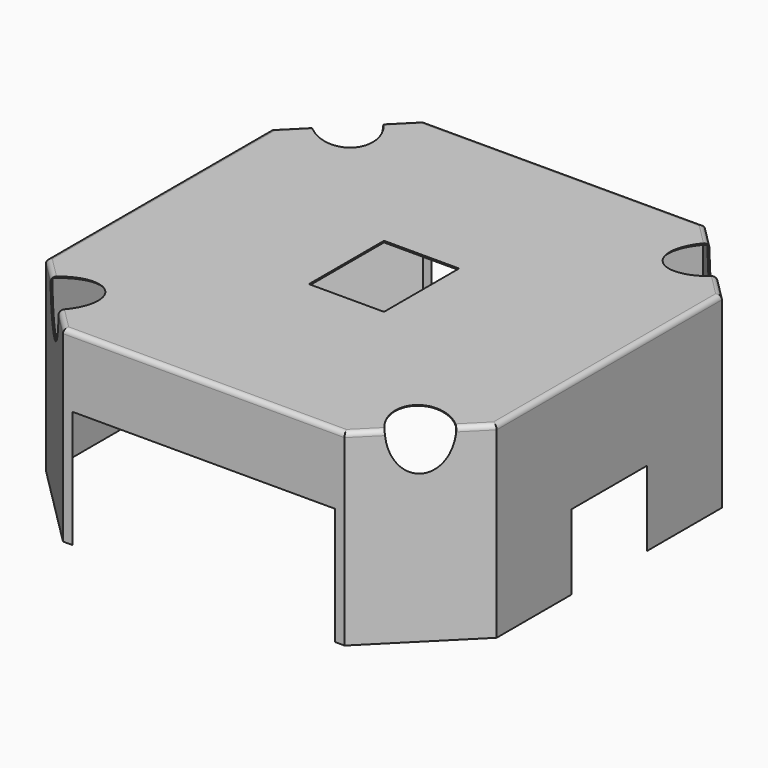
from build123d import *

# Parameters (mm, degrees)
F1_DEPTH       = 240
F2_SIZE        = 90
F3_T           = -1.6
F10_R          = 30
F12_DEPTH      = 78
F11_R          = 30
F13_DEPTH      = 82
F8_R           = 30
F14_DEPTH      = 153
F9_R           = 30
F15_DEPTH      = 141
F17_DEPTH      = 688
F18_W          = 80
F18_H          = 100
F19_DEPTH      = 25
F20_T1_DEPTH   = 325
F20_T3_DEPTH   = 58.6396103068
F20_T5_DEPTH   = 58.6396103068
F20_T7_DEPTH   = 58.6396103068
F20_T9_DEPTH   = 58.6396103068
F20_T11_DEPTH  = 325
F20_T13_DEPTH  = 58.6396103068
F20_T15_DEPTH  = 58.6396103068
F20_T17_DEPTH  = 134.1651513899
F20_T19_DEPTH  = 280
F20_T21_DEPTH  = 89.1651513899
F20_T23_DEPTH  = 100
F20_T29_DEPTH  = 134.1651513899
F20_T33_DEPTH  = 289.1651513899
F20_T40_DEPTH  = 289.1651513899
F20_T44_DEPTH  = 134.1651513899
F20_T51_DEPTH  = 89.1651513899
F20_T55_DEPTH  = 109.1651513899
F20_T62_DEPTH  = 109.1651513899
F20_T66_DEPTH  = 89.1651513899
F20_T73_DEPTH  = 89.1651513899
F20_T77_DEPTH  = 109.1651513899
F20_T84_DEPTH  = 89.1651513899
F20_T88_DEPTH  = 109.1651513899
F20_T95_DEPTH  = 289.1651513899
F20_T99_DEPTH  = 134.1651513899
F20_T106_DEPTH = 134.1651513899
F20_T110_DEPTH = 289.1651513899


# Not quite as in the source:
# - a fillet or chamfer that OpenCascade refuses, or shapes differently, is made with other operations: its cross-section is extruded or revolved along the edge and cut away or added


with BuildPart() as f1:
    # F0 (on Front) → F1 (new body, symmetric)
    with BuildSketch(Plane.XZ):
        Polygon((140, -100), (240, -100), (240, 100), (-240, 100), (-240, -100), (-140, -100), (-140, 25), (140, 25), align=None)
    extrude(amount=F1_DEPTH, both=True)

    # F2
    f2_edges = [f1.edges().sort_by_distance(p)[0] for p in [
        (240, -240, 0),
        (240, 240, 0),
        (-240, 240, 0),
        (-240, -240, 0),
    ]]
    chamfer(f2_edges, length=F2_SIZE)

    # F3
    f3_openings = [f1.faces().sort_by_distance(p)[0] for p in [
        (185.93985, 0, -100),
        (-185.93985, 0, -100),
        (0, 0, 25),
        (140, 0, -37.5),
        (-140, 0, -37.5),
    ]]
    offset(amount=F3_T, openings=f3_openings)

    # F10 (on face) → F12 (cut)
    with BuildSketch(Plane(origin=(-132.8553390593, 132.8553390593, 187.8858223314), x_dir=(0.8660254038, 0.2886751346, 0.4082482905), z_dir=(0.5, -0.5, -0.7071067812))):
        with Locations((-71.7584734456, -101.4818063619)):
            Circle(F10_R)
    extrude(amount=F12_DEPTH, mode=Mode.SUBTRACT)

    # F11 (on face) → F13 (cut)
    with BuildSketch(Plane(origin=(-132.8553390593, -132.8553390593, 187.8858223314), x_dir=(0.8660254038, -0.2886751346, 0.4082482905), z_dir=(-0.5, -0.5, 0.7071067812))):
        with Locations((-71.7584734456, -101.4818063619)):
            Circle(F11_R)
    extrude(amount=-F13_DEPTH, mode=Mode.SUBTRACT)

    # F8 (on face) → F14 (cut)
    with BuildSketch(Plane(origin=(132.8553390593, -132.8553390593, 187.8858223314), x_dir=(0.8660254038, 0.2886751346, -0.4082482905), z_dir=(0.5, -0.5, 0.7071067812))):
        with Locations((71.7584734456, -101.4818063619)):
            Circle(F8_R)
    extrude(amount=-F14_DEPTH, mode=Mode.SUBTRACT)

    # F9 (on face) → F15 (cut)
    with BuildSketch(Plane(origin=(132.8553390593, 132.8553390593, 187.8858223314), x_dir=(0.8660254038, -0.2886751346, -0.4082482905), z_dir=(-0.5, -0.5, -0.7071067812))):
        with Locations((71.7584734456, -101.4818063619)):
            Circle(F9_R)
    extrude(amount=F15_DEPTH, mode=Mode.SUBTRACT)

    # F16 (on face) → F17 (cut)
    with BuildSketch(Plane(origin=(-240, 0, 0), x_dir=(0, -1, 0), z_dir=(-1, 0, 0))):
        Polygon((-50, -20), (-50, -100), (0, -100), (50, -100), (50, -20), align=None)
    extrude(amount=-F17_DEPTH, mode=Mode.SUBTRACT)

    # F18 (on face) → F19 (cut)
    with BuildSketch(Plane.XY.offset(100)):
        Rectangle(F18_W, F18_H)
    extrude(amount=-F19_DEPTH, mode=Mode.SUBTRACT)

    # F20: fillet of radius 5 on 24 edges, made by hand

    # F20_s2 → F20_t1 (cut)
    with BuildSketch(Plane.YZ.offset(-162.5)):
        with BuildLine():
            ThreePointArc((235, 100), (238.5355339059, 98.5355339059), (240, 95))
            Line((240, 95), (240, 100))
            Line((240, 100), (235, 100))
        make_face()
        with BuildLine():
            ThreePointArc((-240, 95), (-238.5355339059, 98.5355339059), (-235, 100))
            Line((-235, 100), (-240, 100))
            Line((-240, 100), (-240, 95))
        make_face()
    extrude(amount=F20_T1_DEPTH, mode=Mode.SUBTRACT)

    # F20_s4 → F20_t3 (cut)
    with BuildSketch(Plane(origin=(12.3743686708, 12.3743686708, 0), x_dir=(0, 0, 1), z_dir=(0.7071067812, 0.7071067812, 0))):
        with BuildLine():
            ThreePointArc((100, -270.7716446628), (98.5355339059, -274.3071785687), (95, -275.7716446628))
            Line((95, -275.7716446628), (100, -275.7716446628))
            Line((100, -275.7716446628), (100, -270.7716446628))
        make_face()
        with BuildLine():
            ThreePointArc((95, 275.7716446628), (98.5355339059, 274.3071785687), (100, 270.7716446628))
            Line((100, 270.7716446628), (100, 275.7716446628))
            Line((100, 275.7716446628), (95, 275.7716446628))
        make_face()
    extrude(amount=F20_T3_DEPTH, mode=Mode.SUBTRACT)

    # F20_s6 → F20_t5 (cut)
    with BuildSketch(Plane(origin=(-12.3743686708, 12.3743686708, 0), x_dir=(0, 0, 1), z_dir=(-0.7071067812, 0.7071067812, 0))):
        with BuildLine():
            ThreePointArc((100, 270.7716446628), (98.5355339059, 274.3071785687), (95, 275.7716446628))
            Line((95, 275.7716446628), (100, 275.7716446628))
            Line((100, 275.7716446628), (100, 270.7716446628))
        make_face()
    extrude(amount=F20_T5_DEPTH, mode=Mode.SUBTRACT)

    # F20_s8 → F20_t7 (cut)
    with BuildSketch(Plane(origin=(53.8388347648, -53.8388347648, 0), x_dir=(0, 0, 1), z_dir=(-0.7071067812, 0.7071067812, 0))):
        with BuildLine():
            ThreePointArc((100, 270.7716446628), (98.5355339059, 274.3071785687), (95, 275.7716446628))
            Line((95, 275.7716446628), (100, 275.7716446628))
            Line((100, 275.7716446628), (100, 270.7716446628))
        make_face()
    extrude(amount=F20_T7_DEPTH, mode=Mode.SUBTRACT)

    # F20_s10 → F20_t9 (cut)
    with BuildSketch(Plane(origin=(-53.8388347648, -53.8388347648, 0), x_dir=(0, 0, 1), z_dir=(0.7071067812, 0.7071067812, 0))):
        with BuildLine():
            ThreePointArc((100, -270.7716446628), (98.5355339059, -274.3071785687), (95, -275.7716446628))
            Line((95, -275.7716446628), (100, -275.7716446628))
            Line((100, -275.7716446628), (100, -270.7716446628))
        make_face()
        with BuildLine():
            ThreePointArc((95, 275.7716446628), (98.5355339059, 274.3071785687), (100, 270.7716446628))
            Line((100, 270.7716446628), (100, 275.7716446628))
            Line((100, 275.7716446628), (95, 275.7716446628))
        make_face()
    extrude(amount=F20_T9_DEPTH, mode=Mode.SUBTRACT)

    # F20_s12 → F20_t11 (cut)
    with BuildSketch(Plane.XZ.offset(-162.5)):
        with BuildLine():
            ThreePointArc((-235, 100), (-238.5355339059, 98.5355339059), (-240, 95))
            Line((-240, 95), (-240, 100))
            Line((-240, 100), (-235, 100))
        make_face()
        with BuildLine():
            ThreePointArc((235, 100), (238.5355339059, 98.5355339059), (240, 95))
            Line((240, 95), (240, 100))
            Line((240, 100), (235, 100))
        make_face()
    extrude(amount=F20_T11_DEPTH, mode=Mode.SUBTRACT)

    # F20_s14 → F20_t13 (cut)
    with BuildSketch(Plane(origin=(-53.8388347648, 53.8388347648, 0), x_dir=(0, 0, 1), z_dir=(0.7071067812, -0.7071067812, 0))):
        with BuildLine():
            ThreePointArc((100, 270.7716446628), (98.5355339059, 274.3071785687), (95, 275.7716446628))
            Line((95, 275.7716446628), (100, 275.7716446628))
            Line((100, 275.7716446628), (100, 270.7716446628))
        make_face()
    extrude(amount=F20_T13_DEPTH, mode=Mode.SUBTRACT)

    # F20_s16 → F20_t15 (cut)
    with BuildSketch(Plane(origin=(12.3743686708, -12.3743686708, 0), x_dir=(0, 0, 1), z_dir=(0.7071067812, -0.7071067812, 0))):
        with BuildLine():
            ThreePointArc((100, 270.7716446628), (98.5355339059, 274.3071785687), (95, 275.7716446628))
            Line((95, 275.7716446628), (100, 275.7716446628))
            Line((100, 275.7716446628), (100, 270.7716446628))
        make_face()
    extrude(amount=F20_T15_DEPTH, mode=Mode.SUBTRACT)

    # F20_s18 → F20_t17 (cut)
    with BuildSketch(Plane.XY.offset(-109.1651513899)):
        with BuildLine():
            ThreePointArc((140, -240), (141.666060556, -238.817424305), (143.666060556, -238.4))
            Line((143.666060556, -238.4), (140, -238.4))
            Line((140, -238.4), (140, -240))
        make_face()
        with BuildLine():
            ThreePointArc((-140, -240), (-141.666060556, -238.817424305), (-143.666060556, -238.4))
            Line((-143.666060556, -238.4), (-140, -238.4))
            Line((-140, -238.4), (-140, -240))
        make_face()
        with BuildLine():
            ThreePointArc((143.666060556, 240), (141.666060556, 239.582575695), (140, 238.4))
            Line((140, 238.4), (140, 240))
            Line((140, 240), (143.666060556, 240))
        make_face()
        with BuildLine():
            ThreePointArc((-143.666060556, 240), (-141.666060556, 239.582575695), (-140, 238.4))
            Line((-140, 238.4), (-140, 240))
            Line((-140, 240), (-143.666060556, 240))
        make_face()
    extrude(amount=F20_T17_DEPTH, mode=Mode.SUBTRACT)

    # F20_s20 → F20_t19 (cut)
    with BuildSketch(Plane.YZ.offset(-140)):
        with BuildLine():
            ThreePointArc((-240, 25), (-238.817424305, 26.666060556), (-238.4, 28.666060556))
            Line((-238.4, 28.666060556), (-238.4, 25))
            Line((-238.4, 25), (-240, 25))
        make_face()
        with BuildLine():
            ThreePointArc((240, 28.666060556), (239.582575695, 26.666060556), (238.4, 25))
            Line((238.4, 25), (240, 25))
            Line((240, 25), (240, 28.666060556))
        make_face()
    extrude(amount=F20_T19_DEPTH, mode=Mode.SUBTRACT)

    # F20_s22 → F20_t21 (cut)
    with BuildSketch(Plane.XY.offset(-109.1651513899)):
        with BuildLine():
            ThreePointArc((-238.4, -53.666060556), (-238.817424305, -51.666060556), (-240, -50))
            Line((-240, -50), (-238.4, -50))
            Line((-238.4, -50), (-238.4, -53.666060556))
        make_face()
        with BuildLine():
            ThreePointArc((-238.4, 53.666060556), (-238.817424305, 51.666060556), (-240, 50))
            Line((-240, 50), (-238.4, 50))
            Line((-238.4, 50), (-238.4, 53.666060556))
        make_face()
        with BuildLine():
            ThreePointArc((240, -50), (238.817424305, -51.666060556), (238.4, -53.666060556))
            Line((238.4, -53.666060556), (238.4, -50))
            Line((238.4, -50), (240, -50))
        make_face()
        with BuildLine():
            ThreePointArc((238.4, 53.666060556), (238.817424305, 51.666060556), (240, 50))
            Line((240, 50), (238.4, 50))
            Line((238.4, 50), (238.4, 53.666060556))
        make_face()
    extrude(amount=F20_T21_DEPTH, mode=Mode.SUBTRACT)

    # F20_s24 → F20_t23 (cut)
    with BuildSketch(Plane.XZ.offset(-50)):
        with BuildLine():
            ThreePointArc((-238.4, -16.333939444), (-238.817424305, -18.333939444), (-240, -20))
            Line((-240, -20), (-238.4, -20))
            Line((-238.4, -20), (-238.4, -16.333939444))
        make_face()
        with BuildLine():
            ThreePointArc((238.4, -16.333939444), (238.817424305, -18.333939444), (240, -20))
            Line((240, -20), (238.4, -20))
            Line((238.4, -20), (238.4, -16.333939444))
        make_face()
    extrude(amount=F20_T23_DEPTH, mode=Mode.SUBTRACT)


with BuildPart() as f20_tool27:
    # F20_s28 → F20_t29 (new body)
    with BuildSketch(Plane.XY.offset(34.1651513899)):
        with BuildLine():
            ThreePointArc((140, -240), (141.666060556, -238.817424305), (143.666060556, -238.4))
            Line((143.666060556, -238.4), (140, -238.4))
            Line((140, -238.4), (140, -240))
        make_face()
    extrude(amount=-F20_T29_DEPTH)

    split(bisect_by=Plane.XY.offset(25), keep=Keep.TOP)


with BuildPart() as f20_tool31:
    # F20_s32 → F20_t33 (new body)
    with BuildSketch(Plane.YZ.offset(-140)):
        with BuildLine():
            ThreePointArc((-240, 25), (-238.817424305, 26.666060556), (-238.4, 28.666060556))
            Line((-238.4, 28.666060556), (-238.4, 25))
            Line((-238.4, 25), (-240, 25))
        make_face()
    extrude(amount=F20_T33_DEPTH)

    split(bisect_by=Plane.YZ.offset(140), keep=Keep.TOP)


with BuildPart() as f20_tool27_1:
    add(f20_tool27.part)

    # F20_t35: intersect F20_tool31
    add(f20_tool31.part, mode=Mode.INTERSECT)


with BuildPart() as f1_1:
    add(f1.part)

    # F20_t25: cut F20_tool27
    add(f20_tool27_1.part, mode=Mode.SUBTRACT)


with BuildPart() as f20_tool38:
    # F20_s39 → F20_t40 (new body)
    with BuildSketch(Plane.YZ.offset(-149.1651513899)):
        with BuildLine():
            ThreePointArc((-240, 25), (-238.817424305, 26.666060556), (-238.4, 28.666060556))
            Line((-238.4, 28.666060556), (-238.4, 25))
            Line((-238.4, 25), (-240, 25))
        make_face()
    extrude(amount=F20_T40_DEPTH)

    split(bisect_by=Plane.YZ.offset(-140), keep=Keep.BOTTOM)


with BuildPart() as f20_tool42:
    # F20_s43 → F20_t44 (new body)
    with BuildSketch(Plane.XY.offset(-100)):
        with BuildLine():
            ThreePointArc((-140, -240), (-141.666060556, -238.817424305), (-143.666060556, -238.4))
            Line((-143.666060556, -238.4), (-140, -238.4))
            Line((-140, -238.4), (-140, -240))
        make_face()
    extrude(amount=F20_T44_DEPTH)

    split(bisect_by=Plane.XY.offset(25), keep=Keep.TOP)


with BuildPart() as f20_tool38_1:
    add(f20_tool38.part)

    # F20_t46: intersect F20_tool42
    add(f20_tool42.part, mode=Mode.INTERSECT)


with BuildPart() as f1_2:
    add(f1_1.part)

    # F20_t36: cut F20_tool38
    add(f20_tool38_1.part, mode=Mode.SUBTRACT)


with BuildPart() as f20_tool49:
    # F20_s50 → F20_t51 (new body)
    with BuildSketch(Plane.XY.offset(-100)):
        with BuildLine():
            ThreePointArc((-238.4, -53.666060556), (-238.817424305, -51.666060556), (-240, -50))
            Line((-240, -50), (-238.4, -50))
            Line((-238.4, -50), (-238.4, -53.666060556))
        make_face()
    extrude(amount=F20_T51_DEPTH)

    split(bisect_by=Plane.XY.offset(-20), keep=Keep.TOP)


with BuildPart() as f20_tool53:
    # F20_s54 → F20_t55 (new body)
    with BuildSketch(Plane.XZ.offset(59.1651513899)):
        with BuildLine():
            ThreePointArc((-238.4, -16.333939444), (-238.817424305, -18.333939444), (-240, -20))
            Line((-240, -20), (-238.4, -20))
            Line((-238.4, -20), (-238.4, -16.333939444))
        make_face()
    extrude(amount=-F20_T55_DEPTH)

    split(bisect_by=Plane.XZ.offset(50), keep=Keep.TOP)


with BuildPart() as f20_tool49_1:
    add(f20_tool49.part)

    # F20_t57: intersect F20_tool53
    add(f20_tool53.part, mode=Mode.INTERSECT)


with BuildPart() as f1_3:
    add(f1_2.part)

    # F20_t47: cut F20_tool49
    add(f20_tool49_1.part, mode=Mode.SUBTRACT)


with BuildPart() as f20_tool60:
    # F20_s61 → F20_t62 (new body)
    with BuildSketch(Plane.XZ.offset(50)):
        with BuildLine():
            ThreePointArc((-238.4, -16.333939444), (-238.817424305, -18.333939444), (-240, -20))
            Line((-240, -20), (-238.4, -20))
            Line((-238.4, -20), (-238.4, -16.333939444))
        make_face()
    extrude(amount=-F20_T62_DEPTH)

    split(bisect_by=Plane.XZ.offset(-50), keep=Keep.BOTTOM)


with BuildPart() as f20_tool64:
    # F20_s65 → F20_t66 (new body)
    with BuildSketch(Plane.XY.offset(-10.8348486101)):
        with BuildLine():
            ThreePointArc((-238.4, 53.666060556), (-238.817424305, 51.666060556), (-240, 50))
            Line((-240, 50), (-238.4, 50))
            Line((-238.4, 50), (-238.4, 53.666060556))
        make_face()
    extrude(amount=-F20_T66_DEPTH)

    split(bisect_by=Plane.XY.offset(-20), keep=Keep.TOP)


with BuildPart() as f20_tool60_1:
    add(f20_tool60.part)

    # F20_t68: intersect F20_tool64
    add(f20_tool64.part, mode=Mode.INTERSECT)


with BuildPart() as f1_4:
    add(f1_3.part)

    # F20_t58: cut F20_tool60
    add(f20_tool60_1.part, mode=Mode.SUBTRACT)


with BuildPart() as f20_tool71:
    # F20_s72 → F20_t73 (new body)
    with BuildSketch(Plane.XY.offset(-10.8348486101)):
        with BuildLine():
            ThreePointArc((240, -50), (238.817424305, -51.666060556), (238.4, -53.666060556))
            Line((238.4, -53.666060556), (238.4, -50))
            Line((238.4, -50), (240, -50))
        make_face()
    extrude(amount=-F20_T73_DEPTH)

    split(bisect_by=Plane.XY.offset(-20), keep=Keep.TOP)


with BuildPart() as f20_tool75:
    # F20_s76 → F20_t77 (new body)
    with BuildSketch(Plane.XZ.offset(-50)):
        with BuildLine():
            ThreePointArc((238.4, -16.333939444), (238.817424305, -18.333939444), (240, -20))
            Line((240, -20), (238.4, -20))
            Line((238.4, -20), (238.4, -16.333939444))
        make_face()
    extrude(amount=F20_T77_DEPTH)

    split(bisect_by=Plane.XZ.offset(50), keep=Keep.TOP)


with BuildPart() as f20_tool71_1:
    add(f20_tool71.part)

    # F20_t79: intersect F20_tool75
    add(f20_tool75.part, mode=Mode.INTERSECT)


with BuildPart() as f1_5:
    add(f1_4.part)

    # F20_t69: cut F20_tool71
    add(f20_tool71_1.part, mode=Mode.SUBTRACT)


with BuildPart() as f20_tool82:
    # F20_s83 → F20_t84 (new body)
    with BuildSketch(Plane.XY.offset(-100)):
        with BuildLine():
            ThreePointArc((238.4, 53.666060556), (238.817424305, 51.666060556), (240, 50))
            Line((240, 50), (238.4, 50))
            Line((238.4, 50), (238.4, 53.666060556))
        make_face()
    extrude(amount=F20_T84_DEPTH)

    split(bisect_by=Plane.XY.offset(-20), keep=Keep.TOP)


with BuildPart() as f20_tool86:
    # F20_s87 → F20_t88 (new body)
    with BuildSketch(Plane.XZ.offset(-59.1651513899)):
        with BuildLine():
            ThreePointArc((238.4, -16.333939444), (238.817424305, -18.333939444), (240, -20))
            Line((240, -20), (238.4, -20))
            Line((238.4, -20), (238.4, -16.333939444))
        make_face()
    extrude(amount=F20_T88_DEPTH)

    split(bisect_by=Plane.XZ.offset(-50), keep=Keep.BOTTOM)


with BuildPart() as f20_tool82_1:
    add(f20_tool82.part)

    # F20_t90: intersect F20_tool86
    add(f20_tool86.part, mode=Mode.INTERSECT)


with BuildPart() as f1_6:
    add(f1_5.part)

    # F20_t80: cut F20_tool82
    add(f20_tool82_1.part, mode=Mode.SUBTRACT)


with BuildPart() as f20_tool93:
    # F20_s94 → F20_t95 (new body)
    with BuildSketch(Plane.YZ.offset(-149.1651513899)):
        with BuildLine():
            ThreePointArc((240, 28.666060556), (239.582575695, 26.666060556), (238.4, 25))
            Line((238.4, 25), (240, 25))
            Line((240, 25), (240, 28.666060556))
        make_face()
    extrude(amount=F20_T95_DEPTH)

    split(bisect_by=Plane.YZ.offset(-140), keep=Keep.BOTTOM)


with BuildPart() as f20_tool97:
    # F20_s98 → F20_t99 (new body)
    with BuildSketch(Plane.XY.offset(-100)):
        with BuildLine():
            ThreePointArc((-143.666060556, 240), (-141.666060556, 239.582575695), (-140, 238.4))
            Line((-140, 238.4), (-140, 240))
            Line((-140, 240), (-143.666060556, 240))
        make_face()
    extrude(amount=F20_T99_DEPTH)

    split(bisect_by=Plane.XY.offset(25), keep=Keep.TOP)


with BuildPart() as f20_tool93_1:
    add(f20_tool93.part)

    # F20_t101: intersect F20_tool97
    add(f20_tool97.part, mode=Mode.INTERSECT)


with BuildPart() as f1_7:
    add(f1_6.part)

    # F20_t91: cut F20_tool93
    add(f20_tool93_1.part, mode=Mode.SUBTRACT)


with BuildPart() as f20_tool104:
    # F20_s105 → F20_t106 (new body)
    with BuildSketch(Plane.XY.offset(34.1651513899)):
        with BuildLine():
            ThreePointArc((143.666060556, 240), (141.666060556, 239.582575695), (140, 238.4))
            Line((140, 238.4), (140, 240))
            Line((140, 240), (143.666060556, 240))
        make_face()
    extrude(amount=-F20_T106_DEPTH)

    split(bisect_by=Plane.XY.offset(25), keep=Keep.TOP)


with BuildPart() as f20_tool108:
    # F20_s109 → F20_t110 (new body)
    with BuildSketch(Plane.YZ.offset(-140)):
        with BuildLine():
            ThreePointArc((240, 28.666060556), (239.582575695, 26.666060556), (238.4, 25))
            Line((238.4, 25), (240, 25))
            Line((240, 25), (240, 28.666060556))
        make_face()
    extrude(amount=F20_T110_DEPTH)

    split(bisect_by=Plane.YZ.offset(140), keep=Keep.TOP)


with BuildPart() as f20_tool104_1:
    add(f20_tool104.part)

    # F20_t112: intersect F20_tool108
    add(f20_tool108.part, mode=Mode.INTERSECT)


with BuildPart() as f1_8:
    add(f1_7.part)

    # F20_t102: cut F20_tool104
    add(f20_tool104_1.part, mode=Mode.SUBTRACT)


solid = f1_8.part
